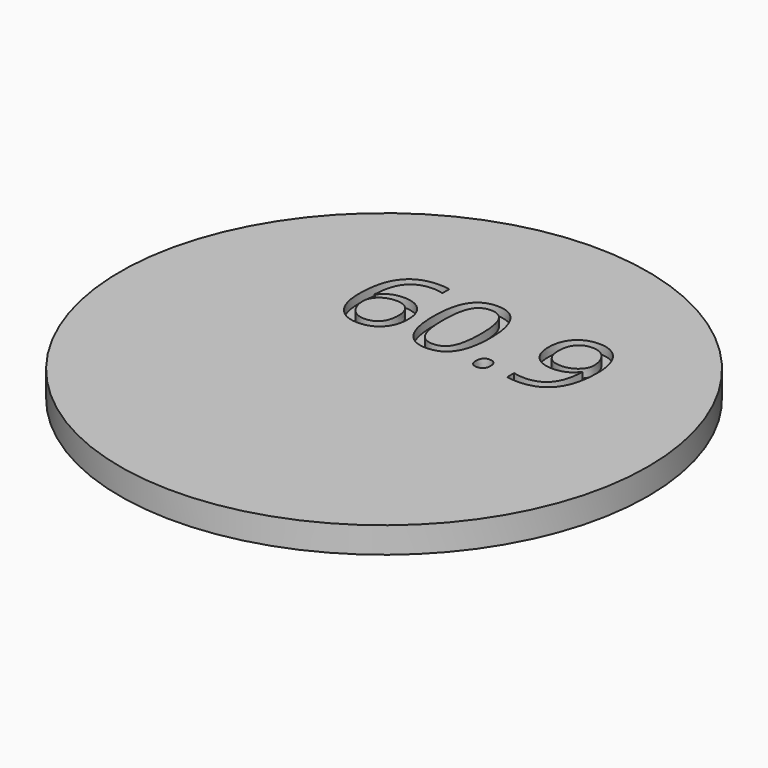
from build123d import *

# Parameters (mm, degrees)
F0_R         = 30.45
F1_DEPTH     = 3
F2_TEXT_SIZE = 14.1389680923
F3_DEPTH     = 1


# Not quite as in the source:
# - Text() gives the source's letters only with a copy of the font that has no kerning and outlines rounded to 1/6400 em; it was checked with that copy


with BuildPart() as f1:
    # F0 (on Top) → F1 (new body)
    with BuildSketch(Plane.XY):
        Circle(F0_R)
    extrude(amount=F1_DEPTH)

    # F2 (on face) → F3 (cut)
    with BuildSketch(Plane.XY.offset(3)):
        with Locations((-11.779778637, 5.7444600388)):
            Text('60.9', F2_TEXT_SIZE, font='Open Sans', text_align=(TextAlign.LEFT, TextAlign.BOTTOM))
    extrude(amount=-F3_DEPTH, mode=Mode.SUBTRACT)


solid = f1.part
